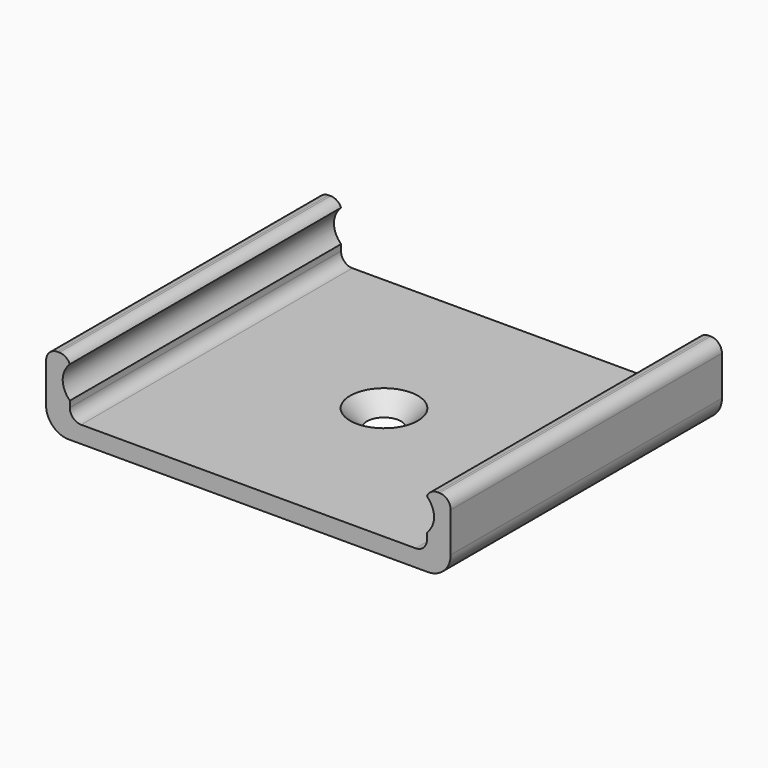
from build123d import *

# Parameters (mm, degrees)
F1_DEPTH       = 30
F3_D           = 3
F3_CSINK_D     = 6
F3_CSINK_ANGLE = 90
F4_DEPTH       = 30.0010001
F5_T1_DEPTH    = 35
F5_T3_DEPTH    = 34.6192422485
F5_T5_DEPTH    = 34.6187341795
F6_R           = 1
F7_R           = 2


# Not quite as in the source:
# - a fillet or chamfer that OpenCascade refuses, or shapes differently, is made with other operations: its cross-section is extruded or revolved along the edge and cut away or added


with BuildPart() as f1:
    # F0 (on Front) → F1 (new body)
    with BuildSketch(Plane.XZ):
        with BuildLine():
            Line((-17.9, 6.5), (-17.9, 0))
            Line((-17.9, 0), (17.9, 0))
            Line((17.9, 0), (17.9, 6.5))
            Line((17.9, 6.5), (15.8, 6.5))
            Line((15.8, 6.5), (15.8, 5.8830036334))
            add(Edge.make_bspline(
                [(15.8, 3.048985269), (17.1972432804, 4.4659944512), (15.8, 5.8830036334)],
                knots=[2.53206789, 2.53206789, 2.53206789, 3.7511174172, 3.7511174172, 3.7511174172], degree=2, weights=[1, 0.8199201727, 1]))
            Line((15.8, 3.048985269), (15.8, 1.5))
            Line((15.8, 1.5), (8, 1.5))
            Line((8, 1.5), (-8, 1.5))
            Line((-8, 1.5), (-15.8, 1.5))
            Line((-15.8, 1.5), (-15.8, 3.0492304381))
            add(Edge.make_bspline(
                [(-16.4293519812, 4.4659944512), (-16.4293519812, 3.687532865), (-15.8, 3.0492304381)],
                knots=[0, 0, 0, 0.6094662657, 0.6094662657, 0.6094662657], degree=2, weights=[1, 0.953927057, 1]))
            add(Edge.make_bspline(
                [(-15.8, 5.8827584643), (-16.4293519812, 5.2444560374), (-16.4293519812, 4.4659944512)],
                knots=[5.6737190415, 5.6737190415, 5.6737190415, 6.2831853072, 6.2831853072, 6.2831853072], degree=2, weights=[1, 0.953927057, 1]))
            Line((-15.8, 5.8827584643), (-15.8, 6.5))
            Line((-15.8, 6.5), (-17.9, 6.5))
        make_face()
        with BuildLine():
            add(Edge.make_bspline(
                [(-15.8, 3.0492304381), (-9.4383519812, -3.4028909356), (-9.4383519812, 4.4659944512), (-9.4383519812, 12.334879838), (-15.8, 5.8827584643)],
                knots=[0.6094662657, 0.6094662657, 0.6094662657, 3.1415926536, 3.1415926536, 5.6737190415, 5.6737190415, 5.6737190415], degree=2, weights=[1, 0.3000386141, 1, 0.3000386141, 1]))
            Line((-15.8, 5.8827584643), (-15.8, 3.0492304381))
        make_face()
        with BuildLine():
            Line((-15.8, 3.0492304381), (-15.8, 5.8827584643))
            add(Edge.make_bspline(
                [(-15.8, 5.8827584643), (-16.4293519812, 5.2444560374), (-16.4293519812, 4.4659944512)],
                knots=[5.6737190415, 5.6737190415, 5.6737190415, 6.2831853072, 6.2831853072, 6.2831853072], degree=2, weights=[1, 0.953927057, 1]))
            add(Edge.make_bspline(
                [(-16.4293519812, 4.4659944512), (-16.4293519812, 3.687532865), (-15.8, 3.0492304381)],
                knots=[0, 0, 0, 0.6094662657, 0.6094662657, 0.6094662657], degree=2, weights=[1, 0.953927057, 1]))
        make_face()
        with BuildLine():
            add(Edge.make_bspline(
                [(15.8, 3.048985269), (17.1972432804, 4.4659944512), (15.8, 5.8830036334)],
                knots=[2.53206789, 2.53206789, 2.53206789, 3.7511174172, 3.7511174172, 3.7511174172], degree=2, weights=[1, 0.8199201727, 1]))
            Line((15.8, 5.8830036334), (15.8, 3.048985269))
        make_face()
        with BuildLine():
            Line((15.8, 3.048985269), (15.8, 5.8830036334))
            add(Edge.make_bspline(
                [(15.8, 5.8830036334), (9.4382216203, 12.3347779991), (9.4382216203, 4.4659944512)],
                knots=[3.7511174172, 3.7511174172, 3.7511174172, 6.2831853072, 6.2831853072, 6.2831853072], degree=2, weights=[1, 0.3000665154, 1]))
            add(Edge.make_bspline(
                [(9.4382216203, 4.4659944512), (9.4382216203, -3.4027890967), (15.8, 3.048985269)],
                knots=[0, 0, 0, 2.53206789, 2.53206789, 2.53206789], degree=2, weights=[1, 0.3000665154, 1]))
        make_face()
    extrude(amount=F1_DEPTH)

    # F3 (through all)
    with Locations(Plane.XY.offset(1.5)):
        with Locations((0, -15)):
            CounterSinkHole(F3_D / 2, F3_CSINK_D / 2, counter_sink_angle=F3_CSINK_ANGLE)

    # F0 (on Front) → F4 (cut, through all)
    with BuildSketch(Plane.XZ):
        with BuildLine():
            Line((15.8, 3.048985269), (15.8, 5.8830036334))
            add(Edge.make_bspline(
                [(15.8, 5.8830036334), (9.4382216203, 12.3347779991), (9.4382216203, 4.4659944512)],
                knots=[3.7511174172, 3.7511174172, 3.7511174172, 6.2831853072, 6.2831853072, 6.2831853072], degree=2, weights=[1, 0.3000665154, 1]))
            add(Edge.make_bspline(
                [(9.4382216203, 4.4659944512), (9.4382216203, -3.4027890967), (15.8, 3.048985269)],
                knots=[0, 0, 0, 2.53206789, 2.53206789, 2.53206789], degree=2, weights=[1, 0.3000665154, 1]))
        make_face()
        with BuildLine():
            add(Edge.make_bspline(
                [(15.8, 3.048985269), (17.1972432804, 4.4659944512), (15.8, 5.8830036334)],
                knots=[2.53206789, 2.53206789, 2.53206789, 3.7511174172, 3.7511174172, 3.7511174172], degree=2, weights=[1, 0.8199201727, 1]))
            Line((15.8, 5.8830036334), (15.8, 3.048985269))
        make_face()
        with BuildLine():
            add(Edge.make_bspline(
                [(-15.8, 3.0492304381), (-9.4383519812, -3.4028909356), (-9.4383519812, 4.4659944512), (-9.4383519812, 12.334879838), (-15.8, 5.8827584643)],
                knots=[0.6094662657, 0.6094662657, 0.6094662657, 3.1415926536, 3.1415926536, 5.6737190415, 5.6737190415, 5.6737190415], degree=2, weights=[1, 0.3000386141, 1, 0.3000386141, 1]))
            Line((-15.8, 5.8827584643), (-15.8, 3.0492304381))
        make_face()
        with BuildLine():
            Line((-15.8, 3.0492304381), (-15.8, 5.8827584643))
            add(Edge.make_bspline(
                [(-15.8, 5.8827584643), (-16.4293519812, 5.2444560374), (-16.4293519812, 4.4659944512)],
                knots=[5.6737190415, 5.6737190415, 5.6737190415, 6.2831853072, 6.2831853072, 6.2831853072], degree=2, weights=[1, 0.953927057, 1]))
            add(Edge.make_bspline(
                [(-16.4293519812, 4.4659944512), (-16.4293519812, 3.687532865), (-15.8, 3.0492304381)],
                knots=[0, 0, 0, 0.6094662657, 0.6094662657, 0.6094662657], degree=2, weights=[1, 0.953927057, 1]))
        make_face()
    extrude(amount=F4_DEPTH, mode=Mode.SUBTRACT)

    # F5: fillet of radius 1 on 4 edges, made by hand

    # F5_s2 → F5_t1 (cut)
    with BuildSketch(Plane.XZ.offset(-2.5)):
        with BuildLine():
            ThreePointArc((-17.9, 5.5), (-17.6071067812, 6.2071067812), (-16.9, 6.5))
            Line((-16.9, 6.5), (-17.9, 6.5))
            Line((-17.9, 6.5), (-17.9, 5.5))
        make_face()
        with BuildLine():
            ThreePointArc((16.9, 6.5), (17.6071067812, 6.2071067812), (17.9, 5.5))
            Line((17.9, 5.5), (17.9, 6.5))
            Line((17.9, 6.5), (16.9, 6.5))
        make_face()
    extrude(amount=F5_T1_DEPTH, mode=Mode.SUBTRACT)

    # F5_s4 → F5_t3 (cut)
    with BuildSketch(Plane.XZ.offset(-2.3096211243)):
        with BuildLine():
            ThreePointArc((-16.7238484497, 6.5), (-16.1683119812, 6.331492172), (-15.8, 5.8827584643))
            Line((-15.8, 5.8827584643), (-15.8, 6.5))
            Line((-15.8, 6.5), (-16.7238484497, 6.5))
        make_face()
    extrude(amount=F5_T3_DEPTH, mode=Mode.SUBTRACT)

    # F5_s6 → F5_t5 (cut)
    with BuildSketch(Plane.XZ.offset(-2.3093670897)):
        with BuildLine():
            ThreePointArc((15.8, 5.8830036334), (16.1683207082, 6.3315658823), (16.7237468359, 6.5))
            Line((16.7237468359, 6.5), (15.8, 6.5))
            Line((15.8, 6.5), (15.8, 5.8830036334))
        make_face()
    extrude(amount=F5_T5_DEPTH, mode=Mode.SUBTRACT)

    # F6
    f6_edges = [f1.edges().sort_by_distance(p)[0] for p in [
        (-15.8, -15, 1.5),
        (15.8, -15, 1.5),
    ]]
    fillet(f6_edges, radius=F6_R)

    # F7
    f7_edges = [f1.edges().sort_by_distance(p)[0] for p in [
        (-17.9, -15, 0),
        (17.9, -15, 0),
    ]]
    fillet(f7_edges, radius=F7_R)


solid = f1.part
